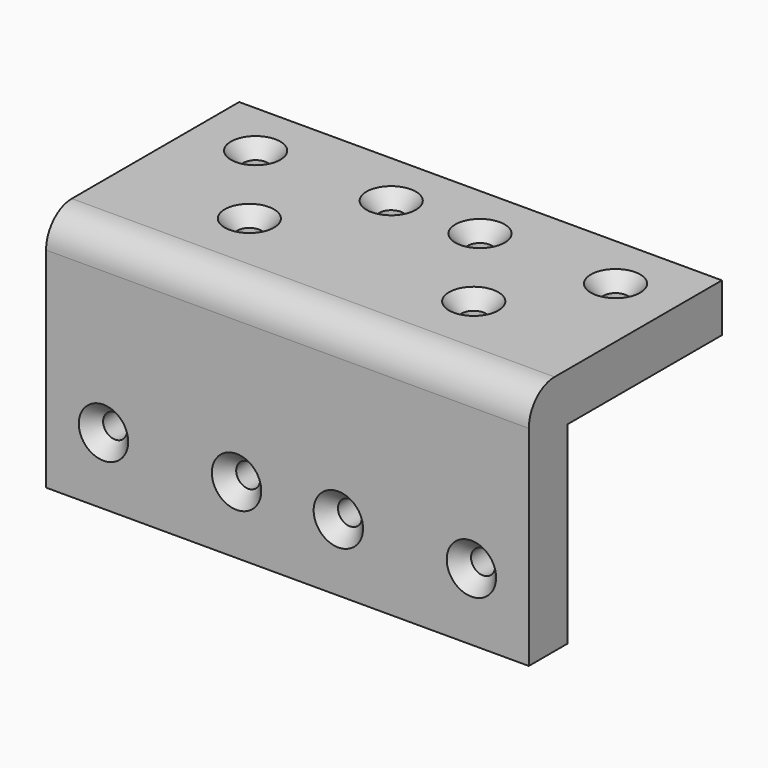
from build123d import *

# Parameters (mm, degrees)
F1_DEPTH       = 38.1
F3_D           = 3.7973
F3_CSINK_D     = 7.7978
F3_CSINK_ANGLE = 82
F4_R           = 5.08
F6_D           = 3.7973
F6_CSINK_D     = 7.7978
F6_CSINK_ANGLE = 82


# Not quite as in the source:
# - a pattern or mirror of a feature is missing from the dataset's text; its kind, count and spacing are read off the source's solid


with BuildPart() as f1:
    # F0 (on Right) → F1 (new body, symmetric)
    with BuildSketch(Plane.YZ):
        Polygon((30.48, 7.62), (-7.62, 7.62), (-7.62, -30.48), (0, -30.48), (0, 0), (30.48, 0), align=None)
    extrude(amount=F1_DEPTH, both=True)

    # F3 (through all)
    with Locations(Plane.XY.offset(7.62)):
        with Locations((-28.405956924, 21.6088658199), (-7.0089674555, 21.6088658199), (-17.7074621897, 6.9944329099)):
            f3 = CounterSinkHole(F3_D / 2, F3_CSINK_D / 2, counter_sink_angle=F3_CSINK_ANGLE)

    # F3_copies: F3 across plane
    add(f3.mirror(Plane(origin=(0, 0, 0), x_dir=(0, 0, 1), z_dir=(1, 0, 0))), mode=Mode.SUBTRACT)

    # F4
    f4_edges = [f1.edges().sort_by_distance(p)[0] for p in [
        (0, -7.62, 7.62),
    ]]
    fillet(f4_edges, radius=F4_R)

    # F6 (through all)
    with Locations(Plane.XZ.offset(7.62)):
        with Locations((-8.0344257876, -19.893276193), (-29.0398038924, -19.893276193)):
            f6 = CounterSinkHole(F6_D / 2, F6_CSINK_D / 2, counter_sink_angle=F6_CSINK_ANGLE)

    # F6_copies: F6 across plane
    add(f6.mirror(Plane(origin=(0, 0, 0), x_dir=(0, 0, 1), z_dir=(1, 0, 0))), mode=Mode.SUBTRACT)


solid = f1.part
